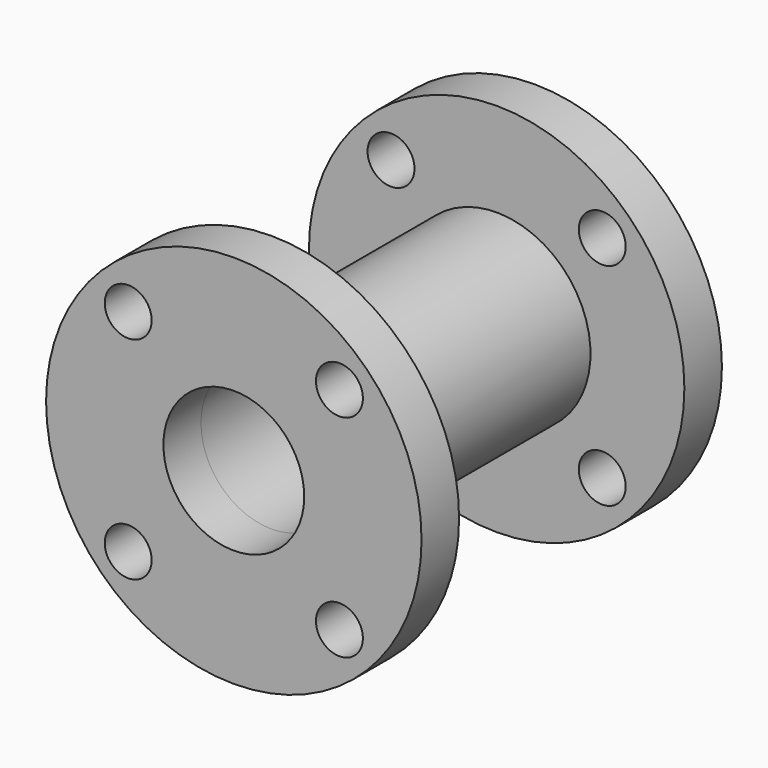
from build123d import *
from build123d import SkipClean  # not in build123d's __all__

# Parameters (mm, degrees)
F0_R     = 50.8
F0_R_2   = 6.35
F0_R_3   = 19.05
F1_DEPTH = 12.7
F2_R     = 25.4
F3_DEPTH = 76.2
F4_R     = 50.8
F4_R_2   = 6.35
F4_R_3   = 19.05
F5_DEPTH = 12.7
F6_R     = 19.05
F7_DEPTH = 76.2


# Not quite as in the source:
# - a feature names something its author has since deleted; it is built from what else it names


with BuildPart() as f1:
    # F0 (on Front) → F1 (new body)
    with BuildSketch(Plane.XZ):
        Circle(F0_R)
        with Locations((-28.575, -28.575)):
            Circle(F0_R_2, mode=Mode.SUBTRACT)
        Circle(F0_R_3, mode=Mode.SUBTRACT)
        with Locations((28.575, -28.575)):
            Circle(F0_R_2, mode=Mode.SUBTRACT)
        with Locations((-28.575, 28.575)):
            Circle(F0_R_2, mode=Mode.SUBTRACT)
        with Locations((28.575, 28.575)):
            Circle(F0_R_2, mode=Mode.SUBTRACT)
    extrude(amount=F1_DEPTH)

    # F2 (on face) → F3 (join)
    with BuildSketch(Plane(origin=(0, 0, 0), x_dir=(-1, 0, 0), z_dir=(0, 1, 0))):
        Circle(F2_R)
    extrude(amount=F3_DEPTH)

    # F4 (on face) → F5 (join)
    with BuildSketch(Plane(origin=(0, 76.2, 0), x_dir=(-1, 0, 0), z_dir=(0, 1, 0))):
        Circle(F4_R)
        with Locations((-28.575, -28.575)):
            Circle(F4_R_2, mode=Mode.SUBTRACT)
        Circle(F4_R_3, mode=Mode.SUBTRACT)
        with Locations((28.575, -28.575)):
            Circle(F4_R_2, mode=Mode.SUBTRACT)
        with Locations((-28.575, 28.575)):
            Circle(F4_R_2, mode=Mode.SUBTRACT)
        with Locations((28.575, 28.575)):
            Circle(F4_R_2, mode=Mode.SUBTRACT)
    extrude(amount=F5_DEPTH)

    # F6 (on face) → F7 (cut)
    with BuildSketch(Plane(origin=(0, 76.2, 0), x_dir=(-1, 0, 0), z_dir=(0, 1, 0))):
        Circle(F6_R)
    with SkipClean():  # cleaning this boolean's faces spoils the solid; the shape is the same uncleaned
        extrude(amount=-F7_DEPTH, mode=Mode.SUBTRACT)


solid = f1.part
